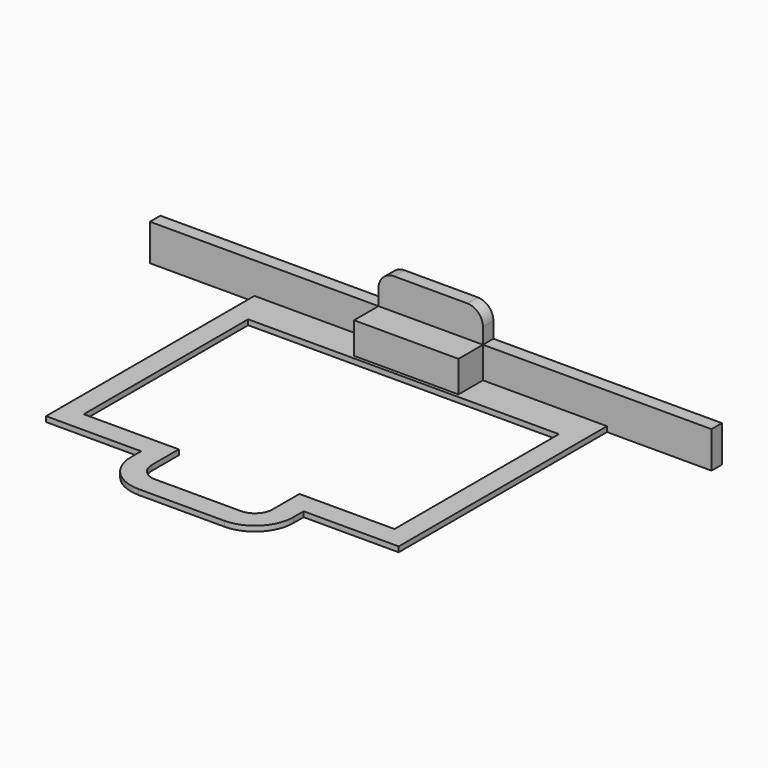
from build123d import *

# Parameters (mm, degrees)
F1_DEPTH      = 100
F0_W          = 2000
F0_H          = 250
F2_DEPTH      = 1200
F2_DEPTH_BACK = 100
F3_DEPTH      = 600
F3_DEPTH_BACK = 100
F0_H_2        = 585
F4_DEPTH      = 600
F4_DEPTH_BACK = 100
F5_R          = 300


with BuildPart() as f1:
    # F0 (on Top) → F1 (new body)
    with BuildSketch(Plane.XY):
        with BuildLine():
            Line((-1000, 0), (-3375, 0))
            Line((-3375, 0), (-3375, -4985))
            Line((-3375, -4985), (-1555, -4985))
            Line((-1555, -4985), (-1555, -5230))
            ThreePointArc((-1555, -5230), (-1339.7234841721, -5749.7234841721), (-820, -5965))
            Line((-820, -5965), (820, -5965))
            ThreePointArc((820, -5965), (1339.7234841721, -5749.7234841721), (1555, -5230))
            Line((1555, -5230), (1555, -4985))
            Line((1555, -4985), (3375, -4985))
            Line((3375, -4985), (3375, 0))
            Line((3375, 0), (1000, 0))
            Line((1000, 0), (1000, -585))
            Line((1000, -585), (-1000, -585))
            Line((-1000, -585), (-1000, 0))
        make_face()
        with BuildLine():
            Line((-2975, -4585), (-2975, -650))
            Line((-2975, -650), (2975, -650))
            Line((2975, -650), (2975, -4585))
            Line((2975, -4585), (1155, -4585))
            Line((1155, -4585), (1155, -5230))
            ThreePointArc((1155, -5230), (1056.8807716975, -5466.8807716975), (820, -5565))
            Line((820, -5565), (-820, -5565))
            ThreePointArc((-820, -5565), (-1056.8807716975, -5466.8807716975), (-1155, -5230))
            Line((-1155, -5230), (-1155, -4585))
            Line((-1155, -4585), (-2975, -4585))
        make_face(mode=Mode.SUBTRACT)
    extrude(amount=-F1_DEPTH)

    # F0 (on Top) → F2 (join, two sides)
    with BuildSketch(Plane.XY) as f2_sk:
        with Locations((0, 125)):
            Rectangle(F0_W, F0_H)
    extrude(amount=F2_DEPTH)
    extrude(f2_sk.sketch, amount=-F2_DEPTH_BACK)

    # F0 (on Top) → F3 (join, two sides)
    with BuildSketch(Plane.XY) as f3_sk:
        Polygon((-5375, 0), (-3375, 0), (-1000, 0), (-1000, 250), (-5375, 250), align=None)
        Polygon((1000, 250), (1000, 0), (3375, 0), (5375, 0), (5375, 250), align=None)
    extrude(amount=F3_DEPTH)
    extrude(f3_sk.sketch, amount=-F3_DEPTH_BACK)

    # F0 (on Top) → F4 (join, two sides)
    with BuildSketch(Plane.XY) as f4_sk:
        with Locations((0, -292.5)):
            Rectangle(F0_W, F0_H_2)
    extrude(amount=F4_DEPTH)
    extrude(f4_sk.sketch, amount=-F4_DEPTH_BACK)

    # F5
    f5_edges = [f1.edges().sort_by_distance(p)[0] for p in [
        (-1000, 125, 1200),
        (1000, 125, 1200),
    ]]
    fillet(f5_edges, radius=F5_R)


solid = f1.part
